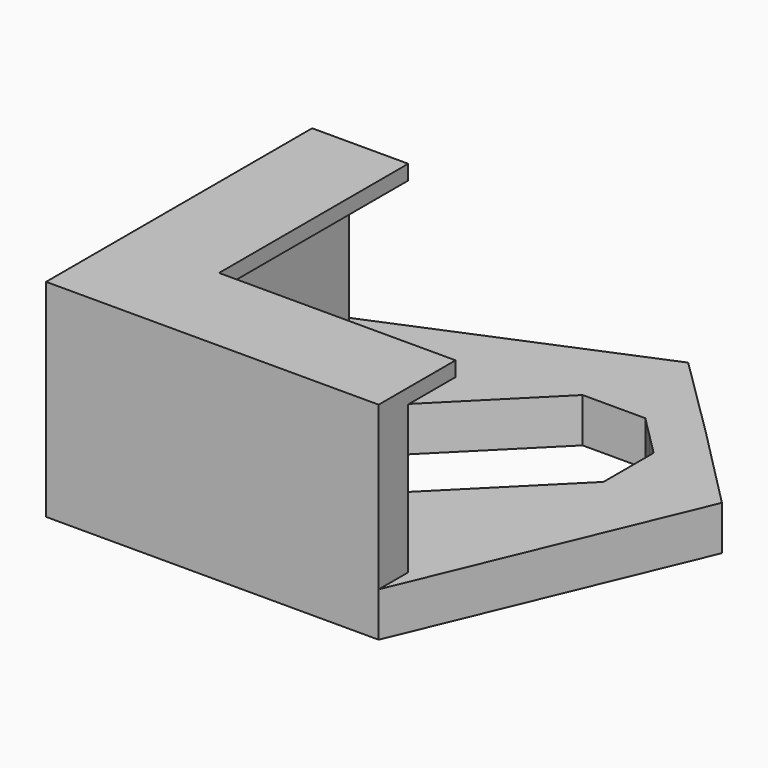
from build123d import *

# Parameters (mm, degrees)
F2_DEPTH  = 7
F4_DEPTH  = 3
F5_DEPTH  = 7
F7_DEPTH  = 1.5
F8_R      = 0.99999
F10_DEPTH = 1


# Not quite as in the source:
# - a fillet or chamfer is up to 0.001 mm smaller than in the source, because OpenCascade refuses the exact size


with BuildPart() as f2:
    # F1 (on offset) → F2 (new body)
    with BuildSketch(Plane.XY.offset(4)):
        Polygon((20, 0), (0, 0), (0, 20), (-2.5, 20), (-2.5, -2.5), (20, -2.5), align=None)
    extrude(amount=F2_DEPTH)



with BuildPart() as f4:
    # F3 (on Top) → F4 (new body)
    with BuildSketch(Plane.XY):
        Polygon((21.591883092, 18.7634559673), (21.591883092, 14.5208152802), (4.5710678119, -2.5), (8.75, -2.5), (20, -2.5), (27.9713179916, 16.5624991059), (22.2989825486, 22.2989889792), (16.5624926754, 27.9713244222), (-2.5, 20), (-2.5, 8.75), (-2.5, 4.5710678119), (14.5208152802, 21.591883092), (18.7634559673, 21.591883092), (20.1776695297, 20.1776695297), align=None)
    extrude(amount=-F4_DEPTH)


with BuildPart() as f2_1:
    add(f2.part)

    add(f4.part)  # F5 merges F4
    # F1 (on offset) → F5 (join)
    with BuildSketch(Plane.XY.offset(4)):
        Polygon((20, 0), (0, 0), (0, 20), (-2.5, 20), (-2.5, -2.5), (20, -2.5), align=None)
    extrude(amount=-F5_DEPTH)

    # F6 (on face) → F7 (join)
    with BuildSketch(Plane(origin=(20.1776695297, 20.1776695297, 0), x_dir=(0.7071067812, -0.7071067812, 0), z_dir=(-0.7071067812, -0.7071067812, 0))):
        with BuildLine():
            Line((-1, -3), (1, -3))
            ThreePointArc((1, -3), (0, -2), (-1, -3))
        make_face()
    extrude(amount=F7_DEPTH)

    # F8 (radius 1 in the source; OpenCascade refuses exactly that, so slightly less here)
    f8_edges = [f2_1.edges().sort_by_distance(p)[0] for p in [
        (19.117009, 19.117009, -2),
    ]]
    fillet(f8_edges, radius=F8_R)

    # F9 (on face) → F10 (join)
    with BuildSketch(Plane.XY.offset(11)):
        Polygon((4, 20), (-2.5, 20), (-2.5, -2.5), (20, -2.5), (20, 4), (4, 4), align=None)
    extrude(amount=-F10_DEPTH)


solid = f2_1.part
